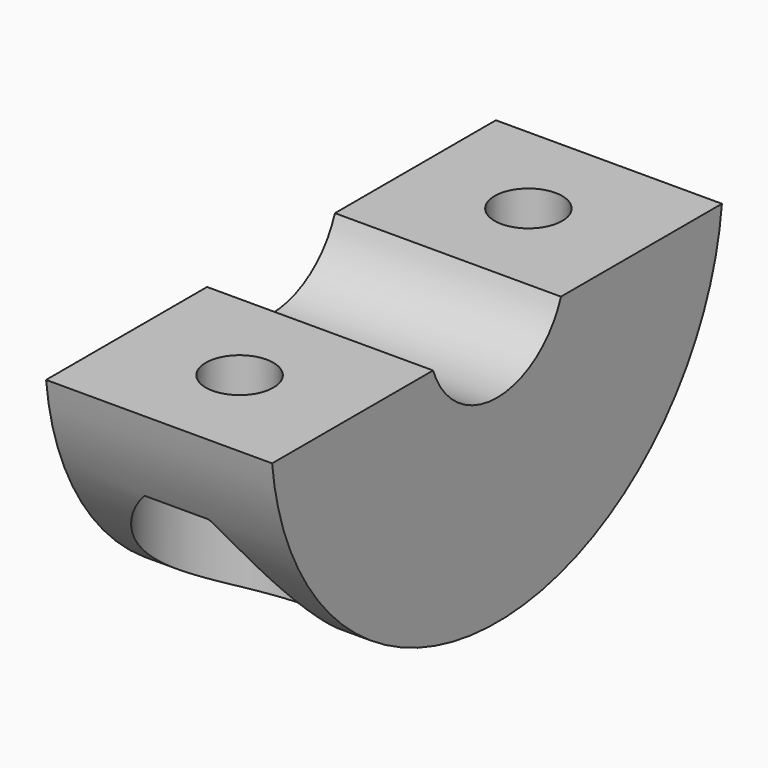
from build123d import *

# Parameters (mm, degrees)
F0_R     = 15.875
F0_R_2   = 4.7625
F1_DEPTH = 12.7
F2_W     = 39.643920958
F2_H     = 19.4333904848
F3_DEPTH = 12.701
F4_R     = 1.89865
F5_DEPTH = 14.2885
F7_R     = 4.7625
F8_DEPTH = 9.525


# Not quite as in the source:
# - a length typed as a fraction of an inch, garbled in the dataset ("3 / 203.2 mm" for 3/8 in), is restored


with BuildPart() as f1:
    # F0 (on Right) → F1 (new body)
    with BuildSketch(Plane.YZ):
        Circle(F0_R)
        Circle(F0_R_2, mode=Mode.SUBTRACT)
    extrude(amount=F1_DEPTH)

    # F2 (on face) → F3 (cut, through all)
    with BuildSketch(Plane.YZ.offset(12.7)):
        with Locations((-1.8631611019, 8.1291952424)):
            Rectangle(F2_W, F2_H)
    extrude(amount=-F3_DEPTH, mode=Mode.SUBTRACT)

    # F4 (on face) → F5 (cut, through all)
    with BuildSketch(Plane.XY.offset(-1.5875)):
        with Locations((6.35, -10.1427768123)):
            Circle(F4_R)
        with Locations((6.35, 10.1427768123)):
            Circle(F4_R)
    extrude(amount=-F5_DEPTH, mode=Mode.SUBTRACT)

    # F7 (on offset) → F8 (cut)
    with BuildSketch(Plane.XY.offset(-15.875)):
        with Locations((6.35, 10.1427768123)):
            Circle(F7_R)
        with Locations((6.35, -10.1427768123)):
            Circle(F7_R)
    extrude(amount=F8_DEPTH, mode=Mode.SUBTRACT)


solid = f1.part
